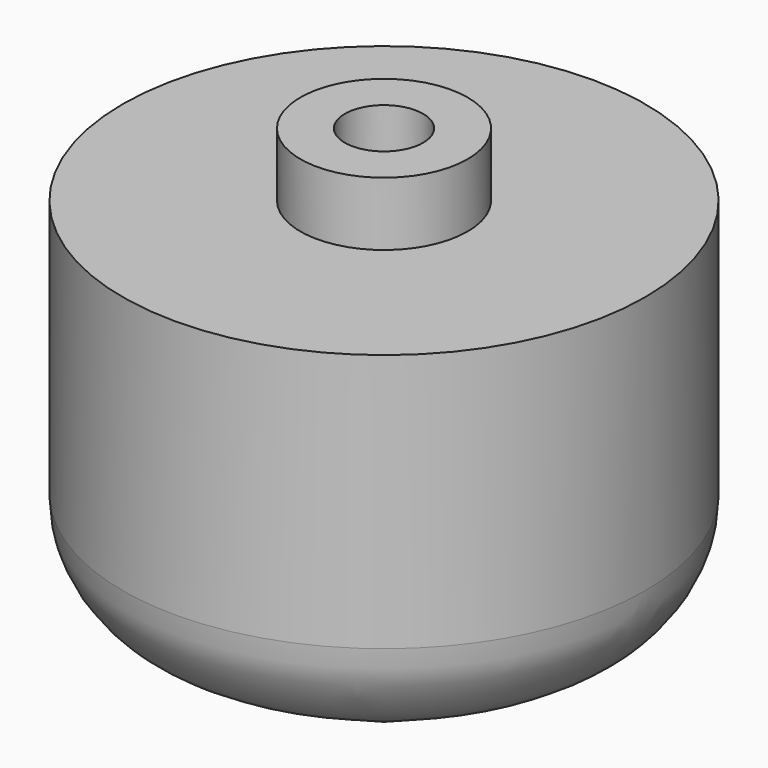
from build123d import *

# Parameters (mm, degrees)
F2_R     = 4.7625
F3_DEPTH = 9.525
F5_R     = 12.7


# Not quite as in the source:
# - the program builds the solid bodies; features that only make, move or delete a surface that nothing else refers to are left out


with BuildPart() as f1:
    # F0 (on Front) → F1 (revolve)
    with BuildSketch(Plane.XZ):
        Polygon((10.16, 55.7645447552), (10.16, 63.5), (0, 63.5), (0, 0), (31.75, 16.6865773499), (31.75, 28.8652195452), (31.75, 46.2049523592), (31.75, 55.7645447552), align=None)
    revolve(axis=Axis((0, 0, 31.75), (0, 0, -1)))

    # F2 (on face) → F3 (cut)
    with BuildSketch(Plane.XY.offset(63.5)):
        Circle(F2_R)
    extrude(amount=-F3_DEPTH, mode=Mode.SUBTRACT)

    # F5
    f5_edges = [f1.edges().sort_by_distance(p)[0] for p in [
        (-31.75, 0, 16.686577),
    ]]
    fillet(f5_edges, radius=F5_R)


solid = f1.part
